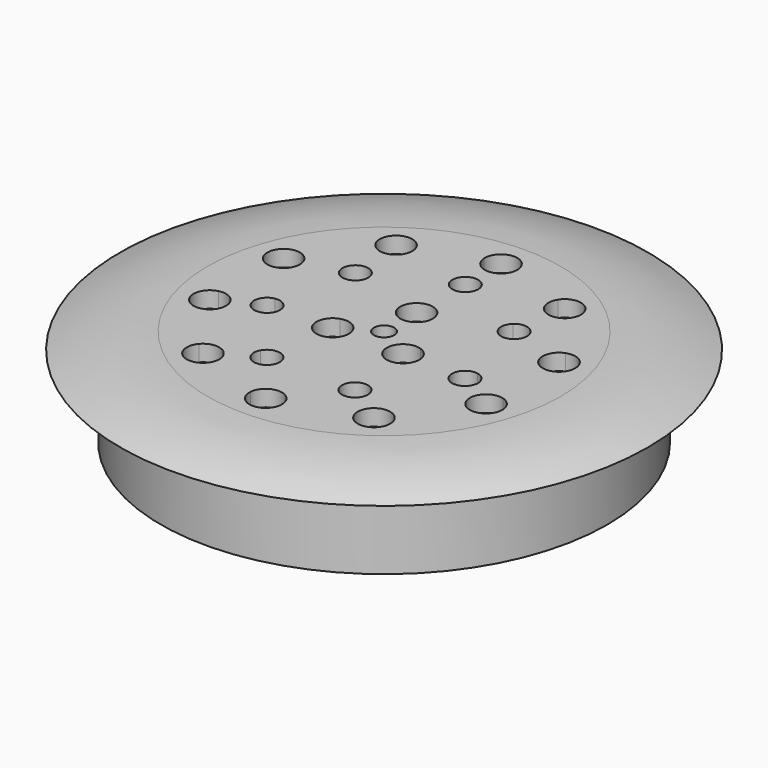
from build123d import *

# Parameters (mm, degrees)
F0_R     = 27.5
F0_R_2   = 25
F1_DEPTH = 10
F2_R     = 32.5
F3_DEPTH = 2
F5_R     = 1.25
F6_DEPTH = 25


# Not quite as in the source:
# - a fillet or chamfer that OpenCascade refuses, or shapes differently, is made with other operations: its cross-section is extruded or revolved along the edge and cut away or added


with BuildPart() as f1:
    # F0 (on Top) → F1 (new body)
    with BuildSketch(Plane.XY):
        Circle(F0_R)
        Circle(F0_R_2, mode=Mode.SUBTRACT)
    extrude(amount=F1_DEPTH)

    # F2 (on face) → F3 (join)
    with BuildSketch(Plane.XY.offset(10)):
        Circle(F2_R)
    extrude(amount=F3_DEPTH)

    # F4: fillet of radius 30 on 1 edges, made by hand

    # F4_s1 → F4_t2 (revolve, cut)
    with BuildSketch(Plane.XZ):
        with BuildLine():
            ThreePointArc((32.5, 10), (27.2068959608, 11.4957624075), (21.7296703857, 12))
            Line((21.7296703857, 12), (32.5, 12))
            Line((32.5, 12), (32.5, 10))
        make_face()
    revolve(axis=Axis((0, 0, 12), (0, 0, 1)), mode=Mode.SUBTRACT)

    # F5 (on face) → F6 (cut)
    with BuildSketch(Plane.XY.offset(12)):
        Circle(F5_R)
        with BuildLine():
            ThreePointArc((16.4249477126, 7.3634973104), (15.2359661654, 4.8852159631), (17.6443655184, 3.5603883849))
            ThreePointArc((17.6443655184, 3.5603883849), (17.1404619361, 5.4958679585), (16.4249477126, 7.3634973104))
        make_face()
        with BuildLine():
            ThreePointArc((16.4249477126, 7.3634973104), (17.1404619361, 5.4958679585), (17.6443655184, 3.5603883849))
            ThreePointArc((17.6443655184, 3.5603883849), (18.7228347058, 4.2727177561), (19.1404619361, 5.4958679585))
            ThreePointArc((19.1404619361, 5.4958679585), (18.273813504, 7.1437496968), (16.4249477126, 7.3634973104))
        make_face()
        with BuildLine():
            ThreePointArc((19.0863675843, -5.6618056107), (18.674651734, -4.4463413126), (17.6090141244, -3.7313029316))
            ThreePointArc((17.6090141244, -3.7313029316), (17.0863675843, -5.6618056107), (16.3527782346, -7.5224094552))
            ThreePointArc((16.3527782346, -7.5224094552), (18.211716708, -7.3151626048), (19.0863675843, -5.6618056107))
        make_face()
        with BuildLine():
            ThreePointArc((16.3527782346, -7.5224094552), (17.0863675843, -5.6618056107), (17.6090141244, -3.7313029316))
            ThreePointArc((17.6090141244, -3.7313029316), (15.1878822972, -5.0327160984), (16.3527782346, -7.5224094552))
        make_face()
        with BuildLine():
            ThreePointArc((8.9296151321, 15.6288826725), (9.4296485775, 12.9260097364), (12.1561268259, 13.2751113213))
            ThreePointArc((12.1561268259, 13.2751113213), (10.6083546497, 14.5417609534), (8.9296151321, 15.6288826725))
        make_face()
        with BuildLine():
            ThreePointArc((8.9296151321, 15.6288826725), (10.6083546497, 14.5417609534), (12.1561268259, 13.2751113213))
            ThreePointArc((12.1561268259, 13.2751113213), (12.491907722, 13.8692820885), (12.6083546497, 14.5417609534))
            ThreePointArc((12.6083546497, 14.5417609534), (11.1751530993, 16.4597649987), (8.9296151321, 15.6288826725))
        make_face()
        with BuildLine():
            ThreePointArc((12.4668572832, -14.6439372647), (12.3536484764, -13.9805979901), (12.0268382899, -13.3923545633))
            ThreePointArc((12.0268382899, -13.3923545633), (10.4668572832, -14.6439372647), (8.7776558162, -15.7147306173))
            ThreePointArc((8.7776558162, -15.7147306173), (11.024350362, -16.5646666749), (12.4668572832, -14.6439372647))
        make_face()
        with BuildLine():
            ThreePointArc((8.7776558162, -15.7147306173), (10.4668572832, -14.6439372647), (12.0268382899, -13.3923545633))
            ThreePointArc((12.0268382899, -13.3923545633), (9.3038731406, -13.0168331242), (8.7776558162, -15.7147306173))
        make_face()
        with BuildLine():
            ThreePointArc((-1.9969111951, 17.8888888889), (0, 16), (1.9969111951, 17.8888888889))
            ThreePointArc((1.9969111951, 17.8888888889), (0, 18), (-1.9969111951, 17.8888888889))
        make_face()
        with BuildLine():
            ThreePointArc((-1.9969111951, 17.8888888889), (0, 18), (1.9969111951, 17.8888888889))
            ThreePointArc((1.9969111951, 17.8888888889), (1.9992276496, 17.944422982), (2, 18))
            ThreePointArc((2, 18), (-0.055577018, 19.9992276496), (-1.9969111951, 17.8888888889))
        make_face()
        with BuildLine():
            ThreePointArc((1.8254698097, -17.9991538471), (1.8249434079, -17.9532699735), (1.8233644798, -17.9074102531))
            ThreePointArc((1.8233644798, -17.9074102531), (-0.1745301903, -17.9991538471), (-2.1702701668, -17.8686856652))
            ThreePointArc((-2.1702701668, -17.8686856652), (-0.2397990464, -19.9980885575), (1.8254698097, -17.9991538471))
        make_face()
        with BuildLine():
            ThreePointArc((-2.1702701668, -17.8686856652), (-0.1745301903, -17.9991538471), (1.8233644798, -17.9074102531))
            ThreePointArc((1.8233644798, -17.9074102531), (-0.155137947, -15.9992478641), (-2.1702701668, -17.8686856652))
        make_face()
        with BuildLine():
            ThreePointArc((-8.3243758543, 14.7447367972), (-8.4009662248, 15.2929114018), (-8.6248712515, 15.7991011104))
            ThreePointArc((-8.6248712515, 15.7991011104), (-10.3243758543, 14.7447367972), (-11.8964190269, 13.5083386964))
            ThreePointArc((-11.8964190269, 13.5083386964), (-9.6701917614, 12.854751831), (-8.3243758543, 14.7447367972))
        make_face()
        with BuildLine():
            ThreePointArc((-11.8964190269, 13.5083386964), (-10.3243758543, 14.7447367972), (-8.6248712515, 15.7991011104))
            ThreePointArc((-8.6248712515, 15.7991011104), (-11.471528727, 16.3830408858), (-11.8964190269, 13.5083386964))
        make_face()
        with BuildLine():
            ThreePointArc((-12.2842724795, -13.1566199934), (-11.9431718341, -16.0424638551), (-9.0807349126, -15.5415653474))
            ThreePointArc((-9.0807349126, -15.5415653474), (-10.7488546507, -14.4382174696), (-12.2842724795, -13.1566199934))
        make_face()
        with BuildLine():
            ThreePointArc((-12.2842724795, -13.1566199934), (-10.7488546507, -14.4382174696), (-9.0807349126, -15.5415653474))
            ThreePointArc((-9.0807349126, -15.5415653474), (-8.8336210518, -15.0143079676), (-8.7488546507, -14.4382174696))
            ThreePointArc((-8.7488546507, -14.4382174696), (-10.0672520016, -12.5579467899), (-12.2842724795, -13.1566199934))
        make_face()
        with BuildLine():
            ThreePointArc((-15.0306668238, 5.827210957), (-15.3718734352, 6.9445311859), (-16.2790713177, 7.6806143657))
            ThreePointArc((-16.2790713177, 7.6806143657), (-17.0306668238, 5.827210957), (-17.5720071839, 3.9018666724))
            ThreePointArc((-17.5720071839, 3.9018666724), (-15.8229169987, 4.2330527591), (-15.0306668238, 5.827210957))
        make_face()
        with BuildLine():
            ThreePointArc((-17.5720071839, 3.9018666724), (-17.0306668238, 5.827210957), (-16.2790713177, 7.6806143657))
            ThreePointArc((-16.2790713177, 7.6806143657), (-18.9229631375, 6.4746788412), (-17.5720071839, 3.9018666724))
        make_face()
        with BuildLine():
            ThreePointArc((-17.6780580424, -3.3891391013), (-19.1032719926, -5.9215706682), (-16.4955729665, -7.2038928718))
            ThreePointArc((-16.4955729665, -7.2038928718), (-17.1929447933, -5.3294136014), (-17.6780580424, -3.3891391013))
        make_face()
        with BuildLine():
            ThreePointArc((-17.6780580424, -3.3891391013), (-17.1929447933, -5.3294136014), (-16.4955729665, -7.2038928718))
            ThreePointArc((-16.4955729665, -7.2038928718), (-15.5505770431, -6.4707409747), (-15.1929447933, -5.3294136014))
            ThreePointArc((-15.1929447933, -5.3294136014), (-15.962137436, -3.7529894043), (-17.6780580424, -3.3891391013))
        make_face()
        with BuildLine():
            ThreePointArc((8.7040688402, 8.9715765407), (8.5293237964, 6.8019087528), (10.6834779133, 6.4894760709))
            ThreePointArc((10.6834779134, 6.4894760709), (9.7728935309, 7.7936225232), (8.7040688402, 8.9715765407))
        make_face()
        with BuildLine():
            ThreePointArc((8.7040688402, 8.9715765407), (9.7728935309, 7.7936225232), (10.6834779134, 6.4894760709))
            ThreePointArc((10.6834779133, 6.4894760709), (11.1832700946, 7.0582315828), (11.3634789221, 7.7936225232))
            ThreePointArc((11.3634789221, 7.7936225232), (10.4170615788, 9.2479297166), (8.7040688402, 8.9715765407))
        make_face()
        with BuildLine():
            ThreePointArc((13.7771842935, -2.7815116745), (13.3979745021, -1.7507202101), (12.4411591434, -1.2114285651))
            ThreePointArc((12.4411591434, -1.2114285651), (12.1865989023, -2.7815116745), (11.7347162243, -4.3065572253))
            ThreePointArc((11.7347162243, -4.3065572253), (13.1382301073, -4.0560154745), (13.7771842935, -2.7815116745))
        make_face()
        with BuildLine():
            ThreePointArc((11.7347162243, -4.3065572253), (12.1865989023, -2.7815116745), (12.4411591434, -1.2114285651))
            ThreePointArc((12.4411591434, -1.2114285651), (10.6358928077, -2.4275731277), (11.7347162243, -4.3065572253))
        make_face()
        with BuildLine():
            ThreePointArc((-1.5873628304, 12.3988015245), (0, 10.9094146088), (1.5873628304, 12.3988015245))
            ThreePointArc((1.5873628304, 12.3988015245), (0, 12.5), (-1.5873628304, 12.3988015245))
        make_face()
        with BuildLine():
            ThreePointArc((-1.5873628304, 12.3988015245), (0, 12.5), (1.5873628304, 12.3988015245))
            ThreePointArc((1.5873628304, 12.3988015245), (1.5897795469, 12.449375114), (1.5905853912, 12.5))
            ThreePointArc((1.5905853912, 12.5), (-0.050624886, 14.0897795469), (-1.5873628304, 12.3988015245))
        make_face()
        with BuildLine():
            ThreePointArc((7.0141321302, -11.2621108488), (6.9622020965, -10.8589960048), (6.8098028583, -10.4822032527))
            ThreePointArc((6.8098028583, -10.4822032527), (5.423546739, -11.2621108488), (3.9494738738, -11.8596650931))
            ThreePointArc((3.9494738738, -11.8596650931), (5.7279503541, -12.8232964002), (7.0141321302, -11.2621108488))
        make_face()
        with BuildLine():
            ThreePointArc((3.9494738738, -11.8596650931), (5.423546739, -11.2621108488), (6.8098028583, -10.4822032527))
            ThreePointArc((6.8098028583, -10.4822032527), (4.733417602, -9.8290429296), (3.9494738738, -11.8596650931))
        make_face()
        with BuildLine():
            ThreePointArc((-8.1823081396, 7.7936225232), (-8.3185863375, 8.4377905712), (-8.7040688402, 8.9715765407))
            ThreePointArc((-8.7040688402, 8.9715765407), (-9.7728935309, 7.7936225232), (-10.6834779134, 6.4894760709))
            ThreePointArc((-10.6834779133, 6.4894760709), (-9.0375025904, 6.3832459595), (-8.1823081396, 7.7936225232))
        make_face()
        with BuildLine():
            ThreePointArc((-10.6834779134, 6.4894760709), (-9.7728935309, 7.7936225232), (-8.7040688402, 8.9715765407))
            ThreePointArc((-8.7040688402, 8.9715765407), (-11.0164632653, 8.7853362936), (-10.6834779133, 6.4894760709))
        make_face()
        with BuildLine():
            ThreePointArc((-6.8098028583, -10.4822032527), (-6.1136758759, -12.695178768), (-3.9494738738, -11.8596650931))
            ThreePointArc((-3.9494738738, -11.8596650931), (-5.423546739, -11.2621108488), (-6.8098028583, -10.4822032527))
        make_face()
        with BuildLine():
            ThreePointArc((-6.8098028583, -10.4822032527), (-5.423546739, -11.2621108488), (-3.9494738738, -11.8596650931))
            ThreePointArc((-3.9494738738, -11.8596650931), (-3.8623611876, -11.5665144639), (-3.8329613478, -11.2621108488))
            ThreePointArc((-3.8329613478, -11.2621108488), (-5.020431895, -9.7234554912), (-6.8098028583, -10.4822032527))
        make_face()
        with BuildLine():
            ThreePointArc((-10.5960135111, -2.7815116745), (-11.1558074379, -1.5701360747), (-12.4411591434, -1.2114285651))
            ThreePointArc((-12.4411591434, -1.2114285651), (-12.1865989023, -2.7815116745), (-11.7347162243, -4.3065572253))
            ThreePointArc((-11.7347162243, -4.3065572253), (-10.9120951022, -3.7331428795), (-10.5960135111, -2.7815116745))
        make_face()
        with BuildLine():
            ThreePointArc((-11.7347162243, -4.3065572253), (-12.1865989023, -2.7815116745), (-12.4411591434, -1.2114285651))
            ThreePointArc((-12.4411591434, -1.2114285651), (-13.7373049969, -3.1354502212), (-11.7347162243, -4.3065572253))
        make_face()
        with BuildLine():
            ThreePointArc((-1.9595917942, 4.6), (0, 3), (1.9595917942, 4.6))
            ThreePointArc((1.9595917942, 4.6), (0, 5), (-1.9595917942, 4.6))
        make_face()
        with BuildLine():
            ThreePointArc((-1.9595917942, 4.6), (0, 5), (1.9595917942, 4.6))
            ThreePointArc((1.9595917942, 4.6), (1.989872306, 4.798982076), (2, 5))
            ThreePointArc((2, 5), (-0.201017924, 6.989872306), (-1.9595917942, 4.6))
        make_face()
        with BuildLine():
            ThreePointArc((6.3301270189, -2.5), (5.9528980242, -1.3309772182), (4.9635127545, -0.6029437252))
            ThreePointArc((4.9635127545, -0.6029437252), (4.3301270189, -2.5), (3.0039209603, -3.9970562748))
            ThreePointArc((3.0039209603, -3.9970562748), (5.1509765431, -4.3237889293), (6.3301270189, -2.5))
        make_face()
        with BuildLine():
            ThreePointArc((3.0039209603, -3.9970562748), (4.3301270189, -2.5), (4.9635127545, -0.6029437252))
            ThreePointArc((4.9635127545, -0.6029437252), (2.5980762114, -1.5), (3.0039209603, -3.9970562748))
        make_face()
        with BuildLine():
            ThreePointArc((-2.3301270189, -2.5), (-3.1611042371, -0.8772289947), (-4.9635127545, -0.6029437252))
            ThreePointArc((-4.9635127545, -0.6029437252), (-4.3301270189, -2.5), (-3.0039209603, -3.9970562748))
            ThreePointArc((-3.0039209603, -3.9970562748), (-2.5063380896, -3.3208495242), (-2.3301270189, -2.5))
        make_face()
        with BuildLine():
            ThreePointArc((-3.0039209603, -3.9970562748), (-4.3301270189, -2.5), (-4.9635127545, -0.6029437252))
            ThreePointArc((-4.9635127545, -0.6029437252), (-6.0621778265, -3.5), (-3.0039209603, -3.9970562748))
        make_face()
    extrude(amount=-F6_DEPTH, mode=Mode.SUBTRACT)


solid = f1.part
